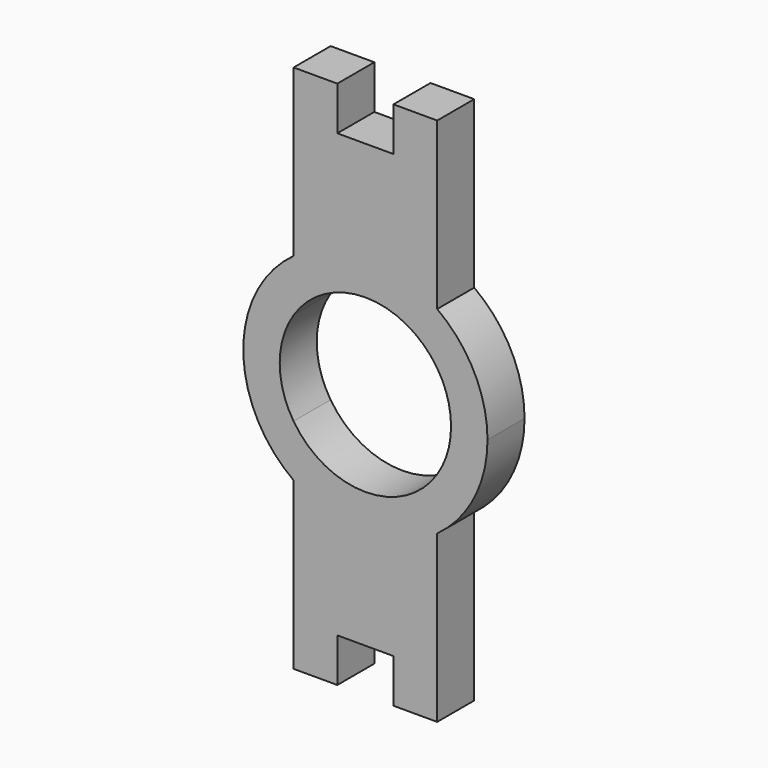
from build123d import *

# Parameters (mm, degrees)
F1_DEPTH = 6.35
F2_W     = 6
F2_H     = 6
F3_DEPTH = 6.35


# Not quite as in the source:
# - a length typed as a fraction of an inch, garbled in the dataset ("3 / 203.2 mm" for 3/8 in), is restored


with BuildPart() as f1:
    # F0 (on Front) → F1 (new body)
    with BuildSketch(Plane.XZ):
        with BuildLine():
            ThreePointArc((9.85, 6.4062469512), (11.2649900133, 3.3410327745), (11.75, 0))
            ThreePointArc((11.75, 0), (11.2649900133, -3.3410327745), (9.85, -6.4062469512))
            Line((9.85, -6.4062469512), (9.85, -13.5476935306))
            ThreePointArc((9.85, -13.5476935306), (14.9256490646, -7.6018089952), (16.75, 0))
            ThreePointArc((16.75, 0), (14.9256490646, 7.6018089952), (9.85, 13.5476935306))
            Line((9.85, 13.5476935306), (9.85, 6.4062469512))
        make_face()
        with BuildLine():
            ThreePointArc((-9.85, 6.4062469512), (0, 11.75), (9.85, 6.4062469512))
            Line((9.85, 6.4062469512), (9.85, 13.5476935306))
            ThreePointArc((9.85, 13.5476935306), (0, 16.75), (-9.85, 13.5476935306))
            Line((-9.85, 13.5476935306), (-9.85, 6.4062469512))
        make_face()
        with BuildLine():
            Line((9.85, -13.5476935306), (9.85, -6.4062469512))
            ThreePointArc((9.85, -6.4062469512), (0, -11.75), (-9.85, -6.4062469512))
            Line((-9.85, -6.4062469512), (-9.85, -13.5476935306))
            ThreePointArc((-9.85, -13.5476935306), (0, -16.75), (9.85, -13.5476935306))
        make_face()
        with BuildLine():
            ThreePointArc((-9.85, -6.4062469512), (-11.75, 0), (-9.85, 6.4062469512))
            Line((-9.85, 6.4062469512), (-9.85, 13.5476935306))
            ThreePointArc((-9.85, 13.5476935306), (-16.75, 0), (-9.85, -13.5476935306))
            Line((-9.85, -13.5476935306), (-9.85, -6.4062469512))
        make_face()
        with BuildLine():
            ThreePointArc((-9.85, 13.5476935306), (0, 16.75), (9.85, 13.5476935306))
            Line((9.85, 13.5476935306), (9.85, 30.31089))
            Line((9.85, 30.31089), (-9.85, 30.31089))
            Line((-9.85, 30.31089), (-9.85, 13.5476935306))
        make_face()
        with BuildLine():
            Line((9.85, -30.31089), (9.85, -13.5476935306))
            ThreePointArc((9.85, -13.5476935306), (0, -16.75), (-9.85, -13.5476935306))
            Line((-9.85, -13.5476935306), (-9.85, -30.31089))
            Line((-9.85, -30.31089), (9.85, -30.31089))
        make_face()
    extrude(amount=F1_DEPTH)

    # F2 (on face) → F3 (join)
    with BuildSketch(Plane.XZ.offset(6.35)):
        with Locations((-6.85, 33.31089)):
            Rectangle(F2_W, F2_H)
        with Locations((6.85, 33.31089)):
            Rectangle(F2_W, F2_H)
        with Locations((-6.85, -33.31089)):
            Rectangle(F2_W, F2_H)
        with Locations((6.85, -33.31089)):
            Rectangle(F2_W, F2_H)
    extrude(amount=-F3_DEPTH)


solid = f1.part
